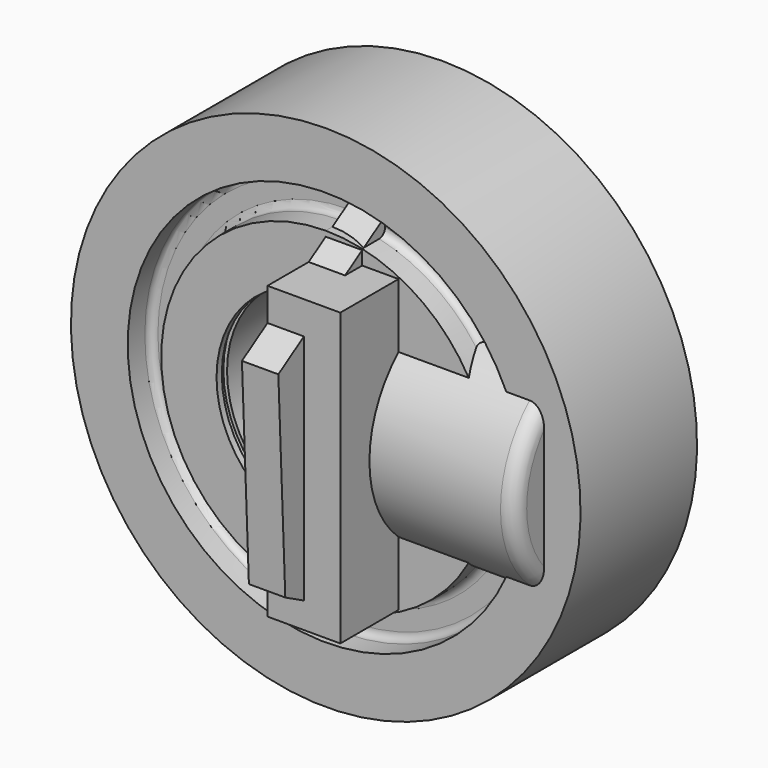
from build123d import *

# Parameters (mm, degrees)
F0_R     = 38.1
F0_R_2   = 12.7
F1_DEPTH = 76.2
F2_R     = 5.08
F4_W     = 101.6
F4_H     = 101.6
F5_DEPTH = 25.4
F7_DEPTH = 12.7


# Not quite as in the source:
# - the program builds the solid bodies; features that only make, move or delete a surface that nothing else refers to are left out


with BuildPart() as f1:
    # F0 (on Right) → F1 (new body)
    with BuildSketch(Plane.YZ):
        Circle(F0_R)
        Circle(F0_R_2, mode=Mode.SUBTRACT)
    extrude(amount=F1_DEPTH)

    # F2
    f2_edges = [f1.edges().sort_by_distance(p)[0] for p in [
        (76.2, -38.1, 0),
        (0, -38.1, 0),
    ]]
    fillet(f2_edges, radius=F2_R)

    # F4 (on Right) → F5 (join)
    with BuildSketch(Plane.YZ):
        Rectangle(F4_W, F4_H)
    extrude(amount=F5_DEPTH)

    # F6 (on Right) → F7 (join)
    with BuildSketch(Plane.YZ):
        Polygon((3.0336469462, -69.7840919279), (61.9516198627, -32.2648306425), (58.9179729165, 37.5192612854), (-3.0336469462, 69.7840919279), (-61.9516198627, 32.2648306425), (-58.9179729165, -37.5192612854), align=None)
    extrude(amount=F7_DEPTH)

    # F8 (on Right) → F9 (revolve)
    with BuildSketch(Plane.YZ):
        with BuildLine():
            Line((25.4, 88.9), (0, 88.9))
            Line((0, 88.9), (-25.4, 88.9))
            Line((-25.4, 88.9), (-25.4, 69.088))
            Line((-25.4, 69.088), (-17.9473628443, 69.088))
            ThreePointArc((-17.9473628443, 69.088), (-16.1513116201, 68.3440512242), (-15.4073628443, 66.548))
            Line((-15.4073628443, 66.548), (-15.4073628443, 59.9419880681))
            ThreePointArc((-15.4073628443, 59.9419880681), (-16.1513116201, 58.1459368439), (-17.9473628443, 57.4019880681))
            Line((-17.9473628443, 57.4019880681), (-25.4, 57.4019880681))
            Line((-25.4, 57.4019880681), (-25.4, 38.1))
            Line((-25.4, 38.1), (-23.114, 38.1))
            Line((-23.114, 38.1), (-23.114, 39.3817271054))
            Line((-23.114, 39.3817271054), (-20.828, 39.3817271054))
            Line((-20.828, 39.3817271054), (-20.828, 38.1))
            Line((-20.828, 38.1), (-1.524, 38.1))
            Line((-1.524, 38.1), (-1.524, 35.56))
            Line((-1.524, 35.56), (0, 35.56))
            Line((0, 35.56), (1.524, 35.56))
            Line((1.524, 35.56), (1.524, 38.1))
            Line((1.524, 38.1), (20.828, 38.1))
            Line((20.828, 38.1), (20.828, 39.3817271054))
            Line((20.828, 39.3817271054), (23.114, 39.3817271054))
            Line((23.114, 39.3817271054), (23.114, 38.1))
            Line((23.114, 38.1), (25.4, 38.1))
            Line((25.4, 38.1), (25.4, 57.4019880681))
            Line((25.4, 57.4019880681), (17.9473628443, 57.4019880681))
            ThreePointArc((17.9473628443, 57.4019880681), (16.1513116201, 58.1459368439), (15.4073628443, 59.9419880681))
            Line((15.4073628443, 59.9419880681), (15.4073628443, 66.548))
            ThreePointArc((15.4073628443, 66.548), (16.1513116201, 68.3440512242), (17.9473628443, 69.088))
            Line((17.9473628443, 69.088), (25.4, 69.088))
            Line((25.4, 69.088), (25.4, 88.9))
        make_face()
    revolve(axis=Axis((0, 12.7, 0), (0, 1, 0)))


solid = f1.part
